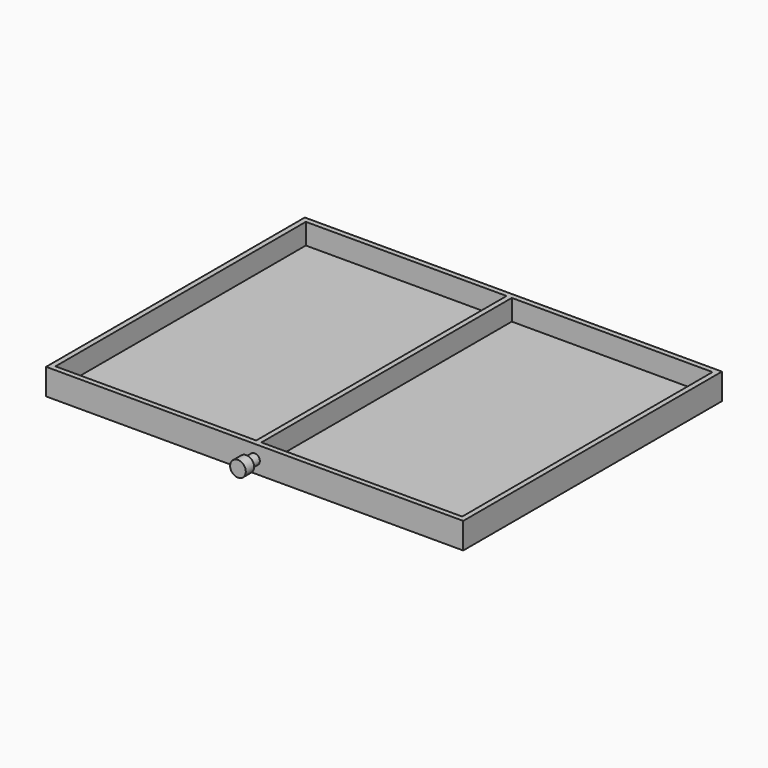
from build123d import *

# Parameters (mm, degrees)
F0_W      = 38.3663107641
F0_H      = 42.2096475959
F1_DEPTH  = 0.6858
F3_W      = 400
F3_H      = 300.087749958
F4_DEPTH  = 5
F5_W      = 5
F5_H      = 300.087749958
F6_DEPTH  = 20
F7_W      = 5
F7_H      = 300.087749958
F8_DEPTH  = 20
F9_W      = 400
F9_H      = 25
F10_DEPTH = 5
F11_W     = 5
F11_H     = 300.087749958
F12_DEPTH = 20
F13_W     = 400
F13_H     = 25
F14_DEPTH = 5
F15_R     = 5
F16_DEPTH = 10
F17_R     = 7.5
F17_R_2   = 5
F18_DEPTH = 10


with BuildPart() as f1:
    # F0 (on Top) → F1 (new body)
    with BuildSketch(Plane.XY):
        with Locations((-14.0401979443, 21.1048237979)):
            Rectangle(F0_W, F0_H)
    extrude(amount=F1_DEPTH)


with BuildPart() as f4:
    # F3 (on Top) → F4 (new body)
    with BuildSketch(Plane.XY):
        Rectangle(F3_W, F3_H)
    extrude(amount=F4_DEPTH)

    # F5 (on face) → F6 (join)
    with BuildSketch(Plane.XY.offset(5)):
        with Locations((-197.5, 0)):
            Rectangle(F5_W, F5_H)
    extrude(amount=F6_DEPTH)

    # F7 (on face) → F8 (join)
    with BuildSketch(Plane.XY.offset(5)):
        with Locations((197.5, 0)):
            Rectangle(F7_W, F7_H)
    extrude(amount=F8_DEPTH)

    # F9 (on face) → F10 (join)
    with BuildSketch(Plane(origin=(0, 150.043874979, 0), x_dir=(-1, 0, 0), z_dir=(0, 1, 0))):
        with Locations((0, 12.5)):
            Rectangle(F9_W, F9_H)
    extrude(amount=F10_DEPTH)

    # F11 (on face) → F12 (join)
    with BuildSketch(Plane.XY.offset(5)):
        Rectangle(F11_W, F11_H)
    extrude(amount=F12_DEPTH)

    # F13 (on face) → F14 (join)
    with BuildSketch(Plane.XZ.offset(150.043874979)):
        with Locations((0, 12.5)):
            Rectangle(F13_W, F13_H)
    extrude(amount=F14_DEPTH)

    # F15 (on face) → F16 (join)
    with BuildSketch(Plane.XZ.offset(155.043874979)):
        with Locations((0, 12.090690434)):
            Circle(F15_R)
    extrude(amount=F16_DEPTH)

    # F17 (on face) → F18 (join)
    with BuildSketch(Plane.XZ.offset(165.043874979)):
        with Locations((0, 12.090690434)):
            Circle(F17_R)
        with Locations((0, 12.090690434)):
            Circle(F17_R_2, mode=Mode.SUBTRACT)
        with Locations((0, 12.090690434)):
            Circle(F17_R_2)
    extrude(amount=F18_DEPTH)


solid = f4.part
